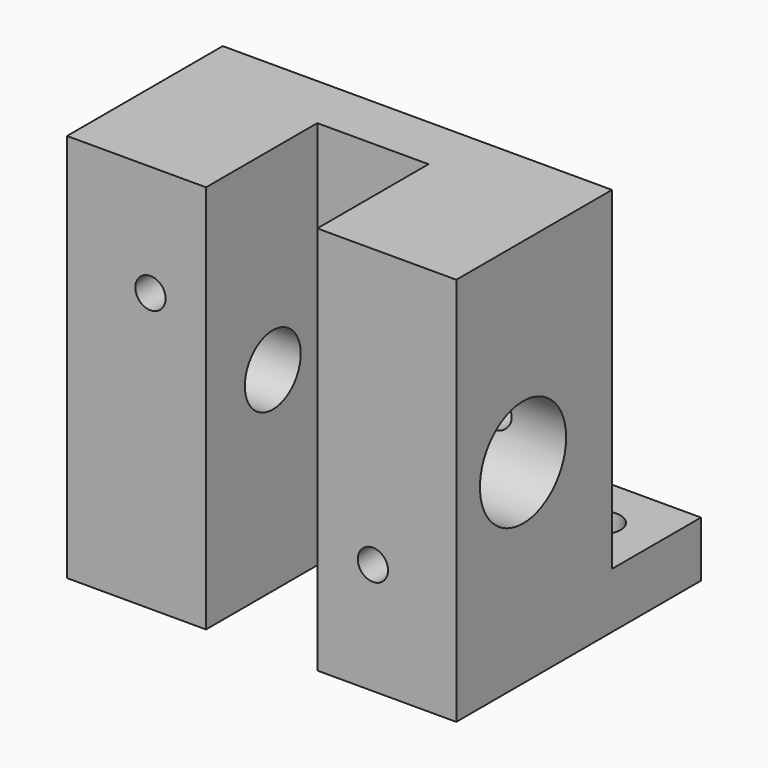
from build123d import *

# Parameters (mm, degrees)
F0_W      = 44.45
F0_H      = 22.225
F1_DEPTH  = 44.45
F2_W      = 12.7
F2_H      = 44.45
F3_DEPTH  = 15.875
F5_W      = 12.7
F5_H      = 6.35
F6_DEPTH  = 12.7
F8_D      = 4.4958
F10_D     = 3.4544
F12_R     = 3.9878
F13_DEPTH = 44.451
F14_R     = 6.15188
F15_DEPTH = 28.575
F17_D     = 3.4544
F17_DEPTH = 12.7
F17_TIP   = 1.0378064612


# Not quite as in the source:
# - an extrude ends at something that could not be found from the text; its depth is read off the source's solid
# - a pattern or mirror of a feature is missing from the dataset's text; its kind, count and spacing are read off the source's solid


with BuildPart() as f1:
    # F0 (on Top) → F1 (new body)
    with BuildSketch(Plane.XY):
        Rectangle(F0_W, F0_H)
    extrude(amount=F1_DEPTH)

    # F2 (on face) → F3 (cut)
    with BuildSketch(Plane.XZ.offset(11.1125)):
        with Locations((0, 22.225)):
            Rectangle(F2_W, F2_H)
    extrude(amount=-F3_DEPTH, mode=Mode.SUBTRACT)

    # F5 (on face) → F6 (join)
    with BuildSketch(Plane(origin=(0, 11.1125, 0), x_dir=(-1, 0, 0), z_dir=(0, 1, 0))):
        with Locations((15.875, 3.175)):
            Rectangle(F5_W, F5_H)
    f6 = extrude(amount=F6_DEPTH)

    # F6_copies: F6 across plane
    add(f6.mirror(Plane(origin=(0, 0, 0), x_dir=(0, 0, 1), z_dir=(1, 0, 0))))

    # F8 (through all)
    with Locations(Plane.XY.offset(6.35)):
        with Locations((-15.875, 17.4625)):
            f8 = Hole(F8_D / 2)

    # F8_copies: F8 across plane
    add(f8.mirror(Plane(origin=(0, 0, 0), x_dir=(0, 0, 1), z_dir=(1, 0, 0))), mode=Mode.SUBTRACT)

    # F10 (through all)
    with Locations(Plane.XZ.offset(11.1125)):
        with Locations((-12.7, 31.75), (12.7, 12.7)):
            Hole(F10_D / 2)

    # F12 (on face) → F13 (cut, through all)
    with BuildSketch(Plane(origin=(-22.225, 0, 0), x_dir=(0, -1, 0), z_dir=(-1, 0, 0))):
        with Locations((1.5875, 22.225)):
            Circle(F12_R)
    extrude(amount=-F13_DEPTH, mode=Mode.SUBTRACT)

    # F14 (on face) → F15 (cut, through all)
    with BuildSketch(Plane.YZ.offset(22.225)):
        with Locations((-1.5875, 22.225)):
            Circle(F14_R)
    extrude(amount=-F15_DEPTH, mode=Mode.SUBTRACT)

    # F17
    with Locations(Plane(origin=(0, 11.1125, 0), x_dir=(-1, 0, 0), z_dir=(0, 1, 0))):
        with Locations((-14.2875, 22.225), (14.2875, 22.225)):
            Hole(F17_D / 2, depth=F17_DEPTH)
            with Locations((0, 0, -(F17_DEPTH + F17_TIP / 2))):  # 118° drill point
                Cone(0, F17_D / 2, F17_TIP, mode=Mode.SUBTRACT)


solid = f1.part
